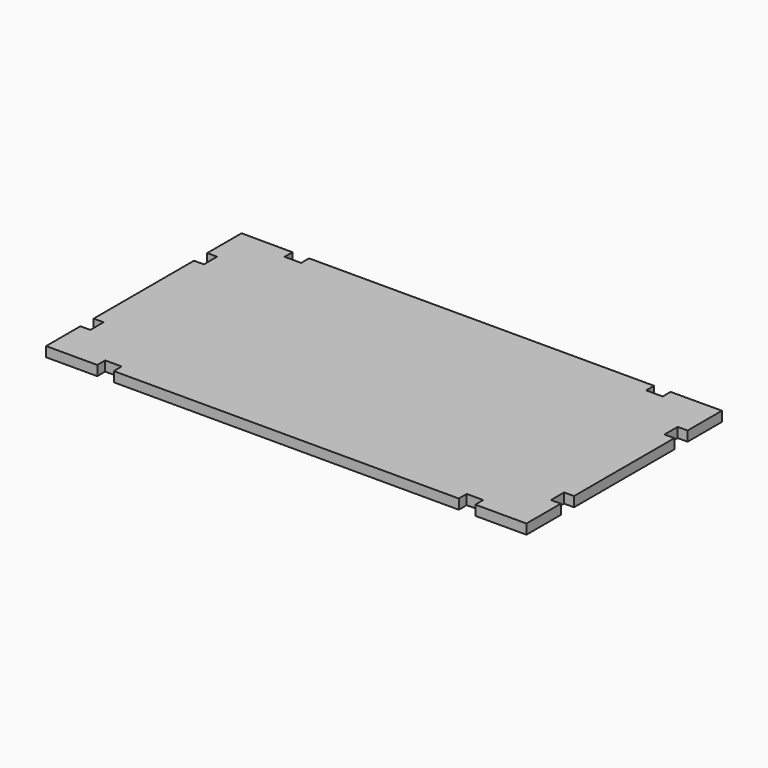
from build123d import *

# Parameters (mm, degrees)
F1_DEPTH = 6


# Not quite as in the source:
# - a feature names something its author has since deleted; it is built from what else it names


with BuildPart() as f1:
    # F0 (on Top) → F1 (new body)
    with BuildSketch(Plane.XY):
        Polygon((-145.5, 69.5100414706), (-145.5, 43.5100414706), (-139.5, 43.5100414706), (-139.5, 33.5100414706), (-145.5, 33.5100414706), (-145.5, -42.4899585294), (-139.5, -42.4899585294), (-139.5, -52.4899585294), (-145.5, -52.4899585294), (-145.5, -78.4899585294), (-114.5, -78.4901820861), (-114.5, -72.4901820861), (-104.5, -72.4901820861), (-104.5, -78.4901820861), (0, -78.4901820861), (104.5, -78.4901820861), (104.5, -72.4901820861), (114.5, -72.4901820861), (114.5, -78.4901820861), (145.5, -78.4899585294), (145.5, -52.4899585294), (139.5, -52.4899585294), (139.5, -42.4899585294), (145.5, -42.4899585294), (145.5, 33.5100414706), (139.5, 33.5100414706), (139.5, 43.5100414706), (145.5, 43.5100414706), (145.5, 69.5100414706), (114.5, 69.3948656799), (114.4997712807, 63.3948656843), (104.5, 63.3948656864), (104.5, 69.3948656864), (0, 69.3948656864), (-104.5, 69.3948656864), (-104.5, 63.3948656864), (-114.4997712807, 63.3948656843), (-114.5, 69.3948656799), align=None)
    extrude(amount=F1_DEPTH)


solid = f1.part
